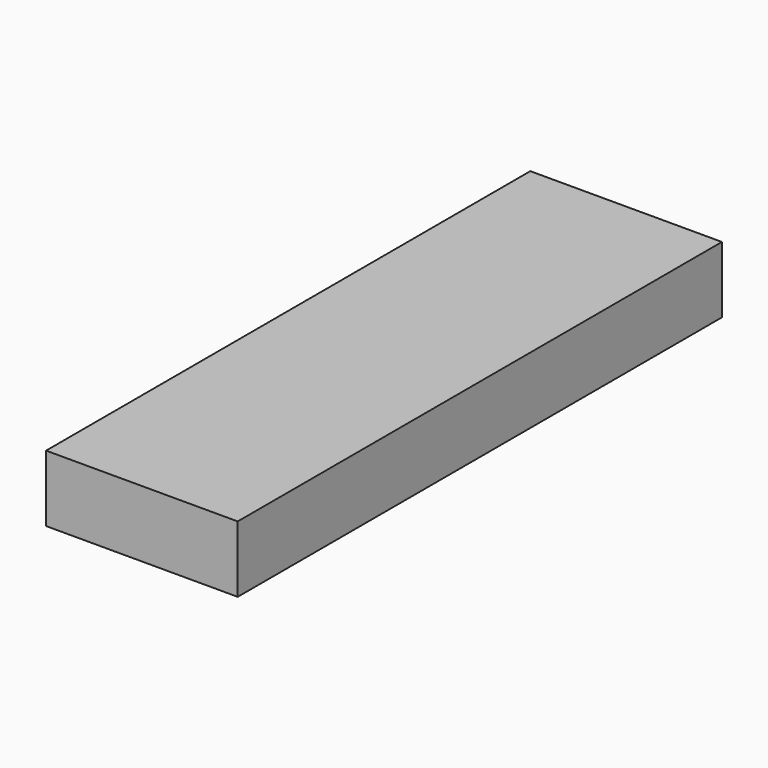
from build123d import *

# Parameters (mm, degrees)
F0_W     = 14.9943903089
F0_H     = 47.3588258028
F1_DEPTH = 5.1970640197


# Not quite as in the source:
# - the program builds the solid bodies; features that only make, move or delete a surface that nothing else refers to are left out


with BuildPart() as f1:
    # F0 (on Top) → F1 (new body)
    with BuildSketch(Plane.XY):
        Rectangle(F0_W, F0_H)
    extrude(amount=F1_DEPTH)


solid = f1.part
